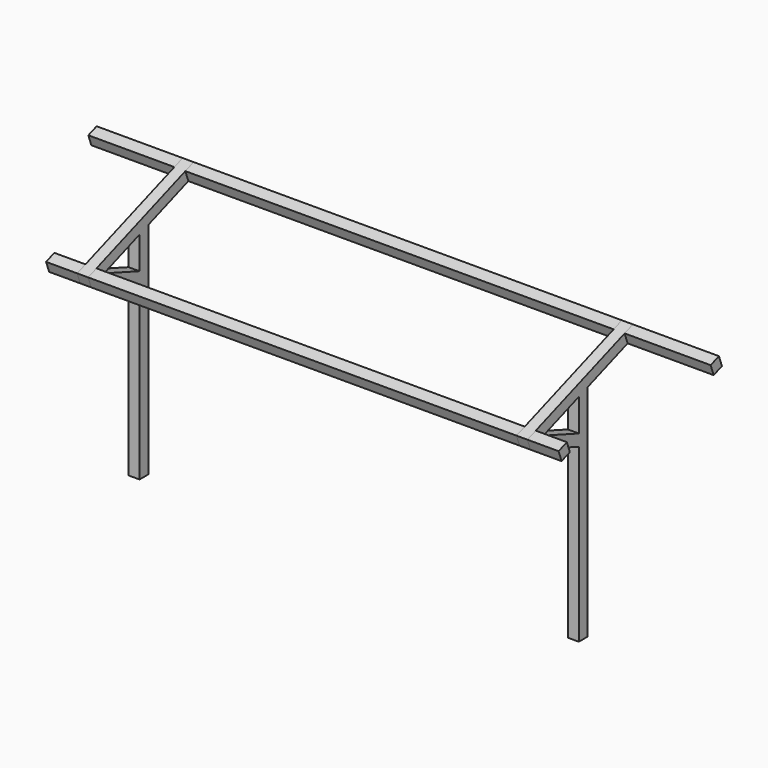
from build123d import *

# Parameters (mm, degrees)
F0_W      = 152.4
F0_H      = 152.4
F1_DEPTH  = 3048
F2_SIZE2  = 55.469054
F2_SIZE   = 152.39999
F3_SIZE2  = 55.469054
F3_SIZE   = 152.39999
F5_DEPTH  = 152.4
F7_W      = 7112
F7_H      = 152.4
F7_W_2    = 8636
F8_DEPTH  = 152.4
F11_DEPTH = 152.4


# Not quite as in the source:
# - a fillet or chamfer is up to 0.001 mm smaller than in the source, because OpenCascade refuses the exact size


with BuildPart() as f1:
    # F0 (on Top) → F1 (new body)
    with BuildSketch(Plane.XY):
        with Locations((-3048, 0)):
            Rectangle(F0_W, F0_H)
    extrude(amount=F1_DEPTH)

    # F3 (size 152.4 and 55.4690637022 in the source; OpenCascade refuses exactly that, so slightly less here)
    f3_edges = [f1.edges().sort_by_distance(p)[0] for p in [
        (-3048, -76.2, 3048),
    ]]
    f3_side = f1.faces().sort_by_distance((-3048, 0, 3048))[0]
    chamfer(f3_edges, length=F3_SIZE, length2=F3_SIZE2, reference=f3_side)

    # F6: F1b across plane


with BuildPart() as f1b:
    # F0 (on Top) → F1, piece 2 (new body)
    with BuildSketch(Plane.XY):
        with Locations((3048, 0)):
            Rectangle(F0_W, F0_H)
    extrude(amount=F1_DEPTH)

    # F2 (size 152.4 and 55.4690637022 in the source; OpenCascade refuses exactly that, so slightly less here)
    f2_edges = [f1b.edges().sort_by_distance(p)[0] for p in [
        (3048, -76.2, 3048),
    ]]
    f2_side = f1b.faces().sort_by_distance((3048, 0, 3048))[0]
    chamfer(f2_edges, length=F2_SIZE, length2=F2_SIZE2, reference=f2_side)

    # F4 (on face) → F5 (join)
    with BuildSketch(Plane.YZ.offset(3124.2)):
        Polygon((-966.5238698428, 2830.6602413437), (-914.4, 2687.4510859359), (-76.1999968818, 2992.5309374328), (76.1999955849, 3047.999998393), (914.4, 3353.0798503619), (862.2761301572, 3496.2890057697), align=None)
    extrude(amount=-F5_DEPTH)


with BuildPart() as f1_1:
    add(f1.part)
    add(f1b.part.mirror(Plane.YZ))


    add(f1b.part)  # F8 merges F1b
    # F7 (on face) → F8 (join)
    with BuildSketch(Plane(origin=(0, -1022.818480288, 2810.170678792), x_dir=(1, 0, 0), z_dir=(0, -0.3420201433, 0.9396926208))):
        with Locations((0, 136.1074731459)):
            Rectangle(F7_W, F7_H)
        with Locations((0, 1929.8757834498)):
            Rectangle(F7_W_2, F7_H)
    extrude(amount=-F8_DEPTH)

    # F9: union 

    # F10 (on face) → F11 (join)
    with BuildSketch(Plane.YZ.offset(3124.2)):
        Polygon((-771.1908445922, 2739.5749557787), (-914.4, 2687.4510859359), (-76.2, 2382.371235574), (-76.2, 2544.5519280993), (-691.6061047076, 2768.5414321986), align=None)
    extrude(amount=-F11_DEPTH)

    # F12: F1 across plane


with BuildPart() as f1_2:
    add(f1_1.part)
    add(f1_1.part.mirror(Plane.YZ))


solid = f1_2.part
